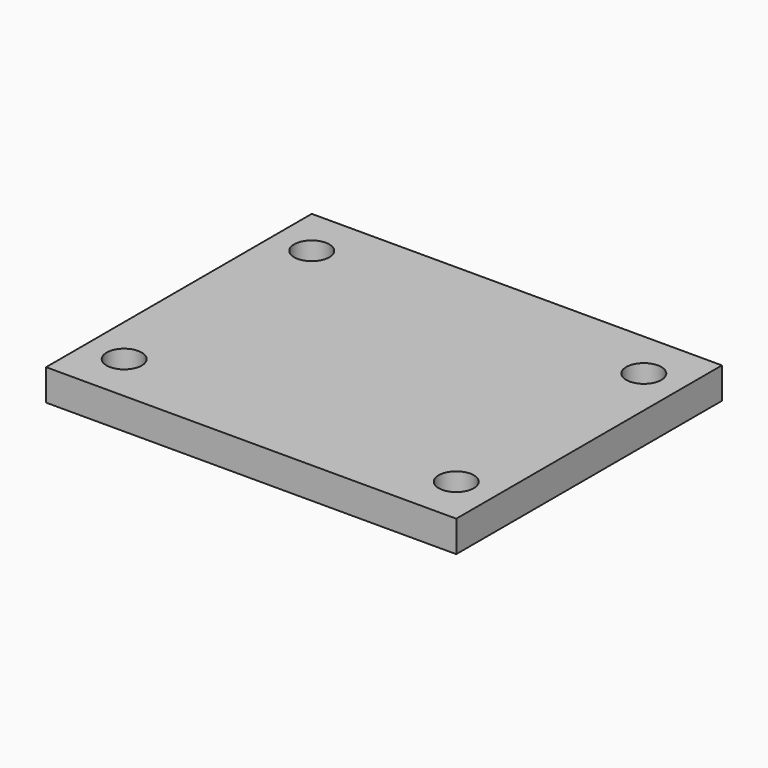
from build123d import *

# Parameters (mm, degrees)
F0_W     = 105
F0_H     = 85
F0_R     = 4
F1_DEPTH = 8
F2_D     = 9
F2_DEPTH = 14
F2_TIP   = 2.7038727856


with BuildPart() as f1:
    # F0 (on Top) → F1 (new body)
    with BuildSketch(Plane.XY):
        Rectangle(F0_W, F0_H)
        with Locations((-42.5, -30)):
            Circle(F0_R, mode=Mode.SUBTRACT)
        with Locations((42.5, -30)):
            Circle(F0_R, mode=Mode.SUBTRACT)
        with Locations((-42.5, 30)):
            Circle(F0_R, mode=Mode.SUBTRACT)
        with Locations((42.5, 30)):
            Circle(F0_R, mode=Mode.SUBTRACT)
        with Locations((-42.5, 30)):
            Circle(F0_R)
        with Locations((42.5, 30)):
            Circle(F0_R)
        with Locations((42.5, -30)):
            Circle(F0_R)
        with Locations((-42.5, -30)):
            Circle(F0_R)
    extrude(amount=F1_DEPTH)

    # F2
    with Locations(Plane(origin=(0, 0, 0), x_dir=(1, 0, 0), z_dir=(0, 0, -1))):
        with Locations((-42.5, -30), (42.5, -30), (42.5, 30), (-42.5, 30)):
            Hole(F2_D / 2, depth=F2_DEPTH)
            with Locations((0, 0, -(F2_DEPTH + F2_TIP / 2))):  # 118° drill point
                Cone(0, F2_D / 2, F2_TIP, mode=Mode.SUBTRACT)


solid = f1.part
